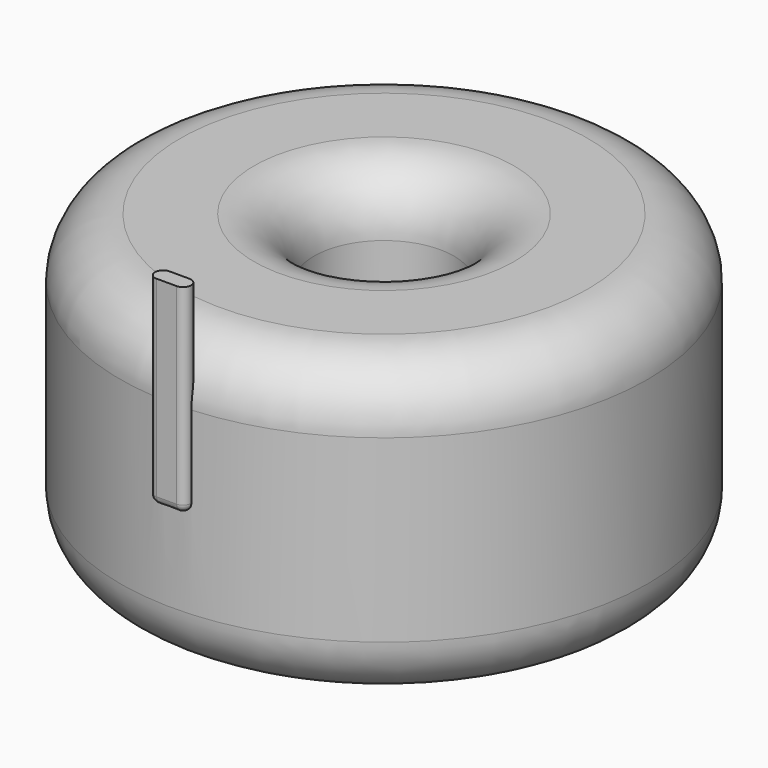
from build123d import *

# Parameters (mm, degrees)
F0_R     = 66
F0_R_2   = 17.5
F1_DEPTH = 37.5
F2_R     = 15
F4_DEPTH = 50
F5_R     = 1.9999


# Not quite as in the source:
# - a fillet or chamfer is up to 0.001 mm smaller than in the source, because OpenCascade refuses the exact size


with BuildPart() as f1:
    # F0 (on Top) → F1 (new body, symmetric)
    with BuildSketch(Plane.XY):
        Circle(F0_R)
        Circle(F0_R_2, mode=Mode.SUBTRACT)
    extrude(amount=F1_DEPTH, both=True)

    # F2
    f2_edges = [f1.edges().sort_by_distance(p)[0] for p in [
        (-17.5, 0, 37.5),
        (17.5, 0, 0),
        (-17.5, 0, -37.5),
        (-66, 0, -37.5),
        (66, 0, 0),
        (-66, 0, 37.5),
    ]]
    fillet(f2_edges, radius=F2_R)

    # F3 (on Top) → F4 (join)
    with BuildSketch(Plane.XY):
        with BuildLine():
            Line((2.5, -63.952634519), (-2.5, -63.952634519))
            ThreePointArc((-2.5, -63.952634519), (-4.5, -65.952634519), (-2.5, -67.952634519))
            Line((-2.5, -67.952634519), (2.5, -67.952634519))
            ThreePointArc((2.5, -67.952634519), (4.5, -65.952634519), (2.5, -63.952634519))
        make_face()
    extrude(amount=F4_DEPTH)

    # F5 (radius 2 in the source; OpenCascade refuses exactly that, so slightly less here)
    f5_edges = [f1.edges().sort_by_distance(p)[0] for p in [
        (0, -67.952635, 0),
    ]]
    fillet(f5_edges, radius=F5_R)


solid = f1.part
